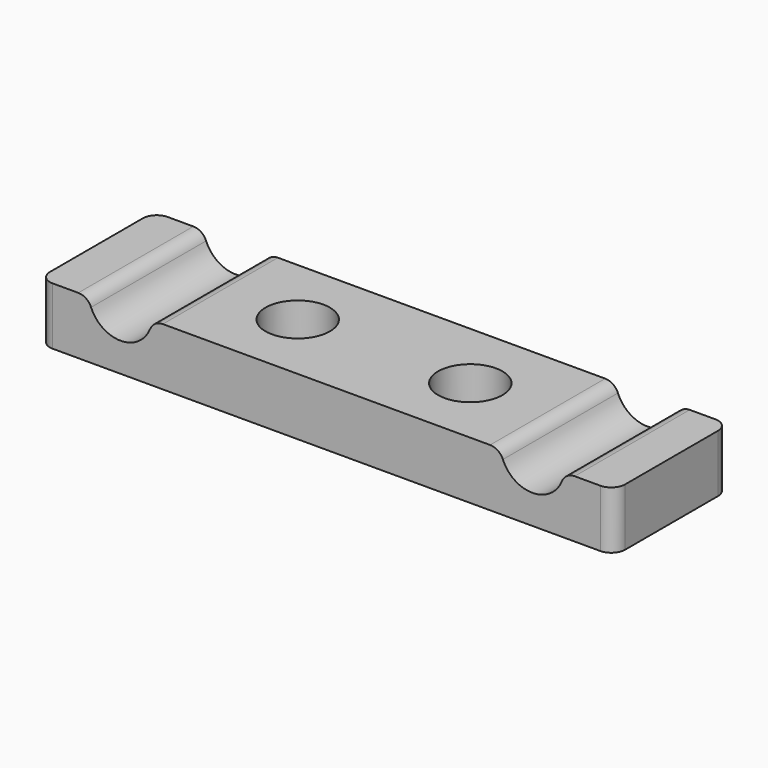
from build123d import *

# Parameters (mm, degrees)
F1_DEPTH = 6.35
F2_R     = 3.5179
F3_DEPTH = 15.876
F4_R     = 1.524
F5_R     = 3.556
F6_DEPTH = 6.35
F8_DEPTH = 1.524


# Not quite as in the source:
# - a pattern or mirror of a feature is missing from the dataset's text; its kind, count and spacing are read off the source's solid


with BuildPart() as f1:
    # F0 (on Top) → F1 (new body)
    with BuildSketch(Plane.XY):
        Polygon((0, 0), (-31.75, 0), (-31.75, -15.875), (0, -15.875), (31.75, -15.875), (31.75, 0), align=None)
    extrude(amount=F1_DEPTH)

    # F2 (on face) → F3 (cut, through all)
    with BuildSketch(Plane(origin=(0, 0, 0), x_dir=(-1, 0, 0), z_dir=(0, 1, 0))):
        with Locations((-22.733, 6.731)):
            Circle(F2_R)
        with Locations((22.733, 6.731)):
            Circle(F2_R)
    extrude(amount=-F3_DEPTH, mode=Mode.SUBTRACT)

    # F4
    f4_edges = [f1.edges().sort_by_distance(p)[0] for p in [
        (31.75, 0, 3.175),
        (31.75, -15.875, 3.175),
        (-31.75, 0, 3.175),
        (-31.75, -15.875, 3.175),
        (19.235793, -7.9375, 6.35),
        (26.230207, -7.9375, 6.35),
        (-26.230207, -7.9375, 6.35),
        (-19.235793, -7.9375, 6.35),
    ]]
    fillet(f4_edges, radius=F4_R)

    # F5 (on face) → F6 (cut, through all)
    with BuildSketch(Plane(origin=(0, 0, 0), x_dir=(1, 0, 0), z_dir=(0, 0, -1))):
        with Locations((-9.525, 7.9375)):
            Circle(F5_R)
    f6 = extrude(amount=-F6_DEPTH, mode=Mode.SUBTRACT)

    # F6_copies: F6 across plane
    add(f6.mirror(Plane(origin=(0, 0, 0), x_dir=(0, 0, 1), z_dir=(1, 0, 0))), mode=Mode.SUBTRACT)

    # F7 (on face) → F8 (cut)
    with BuildSketch(Plane(origin=(0, 0, 0), x_dir=(1, 0, 0), z_dir=(0, 0, -1))):
        Polygon((-9.525, 1.984375), (-6.0879616787, 1.984375), (-2.6509233575, 7.9375), (-6.0879616787, 13.890625), (-9.525, 13.890625), (-12.9620383213, 13.890625), (-16.3990766425, 7.9375), (-12.9620383213, 1.984375), align=None)
    f8 = extrude(amount=-F8_DEPTH, mode=Mode.SUBTRACT)

    # F8_copies: F8 across plane
    add(f8.mirror(Plane(origin=(0, 0, 0), x_dir=(0, 0, 1), z_dir=(1, 0, 0))), mode=Mode.SUBTRACT)


solid = f1.part
